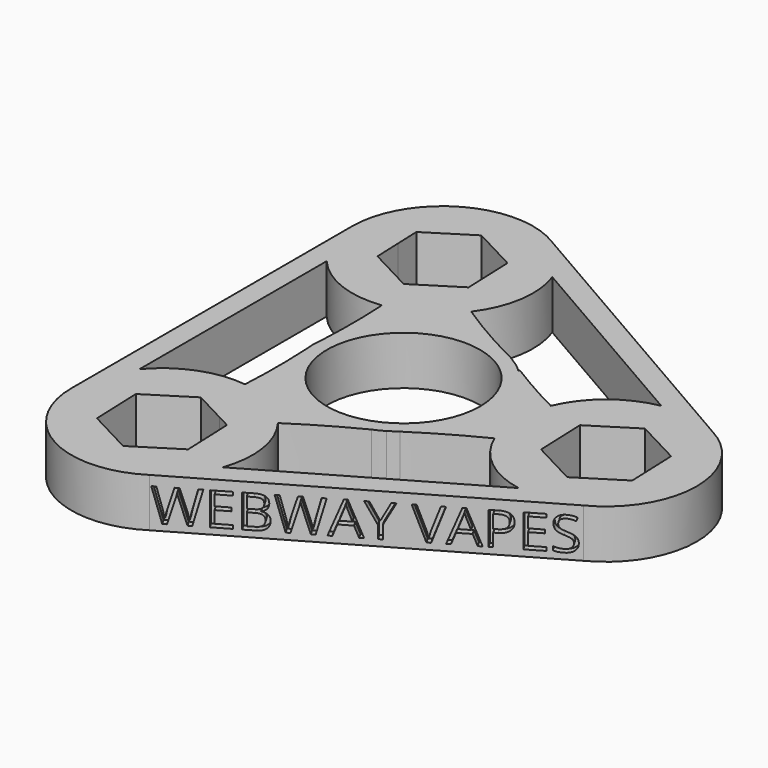
from build123d import *

# Parameters (mm, degrees)
F0_R         = 11
F1_DEPTH     = 7
F2_TEXT_SIZE = 6.7022724893
F3_DEPTH     = 1
F4_TEXT_SIZE = 6.5682270395
F5_DEPTH     = 1
F6_TEXT_SIZE = 6.5682270395
F7_DEPTH     = 1


# Not quite as in the source:
# - Text() gives the source's letters only with a copy of the font that has no kerning and outlines rounded to 1/6400 em; it was checked with that copy


with BuildPart() as f1:
    # F0 (on Top) → F1 (new body)
    with BuildSketch(Plane.XY):
        with BuildLine():
            ThreePointArc((-7.6287234995, 36.1940918561), (-20.8266237724, 36.5516209861), (-27.530946799, 25.1777715301))
            Line((-27.530946799, 25.1777715301), (-27.530946799, -25.1833324685))
            ThreePointArc((-27.530946799, -25.1833324685), (-20.7784207232, -36.5837302495), (-7.5357053272, -36.1408229088))
            Line((-7.5357053272, -36.1408229088), (35.0748929735, -11.5395825096))
            ThreePointArc((35.0748929735, -11.5395825096), (42.0829321515, -0.0578107695), (35.1723502351, 11.4828804138))
            Line((35.1723502351, 11.4828804138), (-7.6287234995, 36.1940918561))
        make_face()
        with Locations((-14.530946799, -25.1833324685)):
            Circle(F0_R, mode=Mode.SUBTRACT)
        with BuildLine():
            ThreePointArc((-12.9255685554, 12.277276939), (-12.7675398796, 6.9299853313), (-12.9033720663, 1.5820838534))
            ThreePointArc((-12.9033720663, 1.5820838534), (-6.4302872117, 11.2982921884), (5.2290918379, 11.9019577613))
            ThreePointArc((5.2290918379, 11.9019577613), (0.4581302885, 14.4888211029), (-4.1613203284, 17.3374369162))
            ThreePointArc((-4.1613203284, 17.3374369162), (-1.6796615961, 23.2170398726), (-2.2951140053, 29.5691717447))
            Line((-2.2951140053, 29.5691717447), (26.7681963735, 12.7894616739))
            ThreePointArc((26.7681963735, 12.7894616739), (20.9564789287, 10.144084315), (17.1054325569, 5.0506058502))
            ThreePointArc((17.1054325569, 5.0506058502), (13.0262022486, 7.2270838071), (9.054869709, 9.5947185056))
            Line((9.054869709, 9.5947185056), (8.948459988, 9.4300086873))
            ThreePointArc((8.948459988, 9.4300086873), (11.9442450545, 5.1317648113), (13, 0))
            ThreePointArc((13, 0), (11.62464331, -5.8195934493), (7.7895895515, -10.4077997011))
            ThreePointArc((7.7895895515, -10.4077997011), (12.3729190289, -7.6017999865), (17.104052334, -5.0528941141))
            ThreePointArc((17.104052334, -5.0528941141), (20.9524134175, -10.1463878699), (26.761439255, -12.7937980177))
            Line((26.761439255, -12.7937980177), (-2.2927959761, -29.5682685494))
            ThreePointArc((-2.2927959761, -29.5682685494), (-1.6817089539, -23.2092284187), (-4.173509012, -17.3269030958))
            ThreePointArc((-4.173509012, -17.3269030958), (0.3360289764, -14.5406855904), (4.9904853555, -12.0039600098))
            ThreePointArc((4.9904853555, -12.0039600098), (-6.6086120064, -11.1949206049), (-12.9210698593, -1.4303683763))
            ThreePointArc((-12.9210698593, -1.4303683763), (-12.7767748148, -6.8562127832), (-12.9349879797, -12.2816691863))
            ThreePointArc((-12.9349879797, -12.2816691863), (-19.2689540032, -13.0774955402), (-24.4604024316, -16.7925094551))
            Line((-24.4604024316, -16.7925094551), (-24.4604024316, 16.7869485168))
            ThreePointArc((-24.4604024316, 16.7869485168), (-19.2645342894, 13.0702057355), (-12.9255685554, 12.277276939))
        make_face(mode=Mode.SUBTRACT)
        with BuildLine():
            ThreePointArc((-25.530946799, 25.1777715301), (-14.530946799, 36.1777715301), (-3.530946799, 25.1777715301))
            ThreePointArc((-3.530946799, 25.1777715301), (-14.530946799, 14.1777715301), (-25.530946799, 25.1777715301))
        make_face(mode=Mode.SUBTRACT)
        with Locations((29.0830486264, -0.0027804692)):
            Circle(F0_R, mode=Mode.SUBTRACT)
        with BuildLine():
            ThreePointArc((-12.9033720663, 1.5820838534), (-12.9484673329, 0.7908453402), (-13, 0))
            ThreePointArc((-13, 0), (-12.9997736844, -0.0767082424), (-12.9990947455, -0.153413814))
            ThreePointArc((-12.9990947455, -0.153413814), (-12.9579854367, -0.7917629718), (-12.9210698593, -1.4303683763))
            ThreePointArc((-12.9210698593, -1.4303683763), (-6.6086120064, -11.1949206049), (4.9904853555, -12.0039600098))
            ThreePointArc((4.9904853555, -12.0039600098), (5.7761571729, -11.6462873189), (6.5363588729, -11.2372600168))
            ThreePointArc((6.5363588729, -11.2372600168), (7.1613741873, -10.8201123831), (7.7895895515, -10.4077997011))
            ThreePointArc((7.7895895515, -10.4077997011), (11.62464331, -5.8195934493), (13, 0))
            ThreePointArc((13, 0), (11.9442450545, 5.1317648113), (8.948459988, 9.4300086873))
            ThreePointArc((8.948459988, 9.4300086873), (8.4010552812, 9.9207998751), (7.8267807235, 10.3798604762))
            ThreePointArc((7.8267807235, 10.3798604762), (7.1580547417, 10.8183902406), (6.4929522165, 11.2623963486))
            ThreePointArc((6.4929522165, 11.2623963486), (6.4256273814, 11.3009430029), (6.3580737149, 11.3390872047))
            ThreePointArc((6.3580737149, 11.3390872047), (5.7926713707, 11.618694424), (5.2290918379, 11.9019577613))
            ThreePointArc((5.2290918379, 11.9019577613), (-6.4302872117, 11.2982921884), (-12.9033720663, 1.5820838534))
        make_face()
        with BuildLine():
            ThreePointArc((-11, 0), (0, 11), (11, 0))
            ThreePointArc((11, 0), (0, -11), (-11, 0))
        make_face(mode=Mode.SUBTRACT)
        with Locations((-14.530946799, -25.1833324685)):
            Circle(F0_R)
        Polygon((-21.0194197971, -21.7682114622), (-14.8176017496, -17.8565895173), (-10.2373305753, -20.2673540079), (-8.3291287516, -21.2717105235), (-8.042473801, -28.5984534747), (-14.2442918485, -32.5100754196), (-17.1564293953, -30.9773107596), (-20.7327648465, -29.0949544134), align=None, mode=Mode.SUBTRACT)
        with BuildLine():
            ThreePointArc((-25.530946799, 25.1777715301), (-14.530946799, 14.1777715301), (-3.530946799, 25.1777715301))
            ThreePointArc((-3.530946799, 25.1777715301), (-14.530946799, 36.1777715301), (-25.530946799, 25.1777715301))
        make_face()
        Polygon((-20.7457503175, 21.2642133583), (-20.8988662153, 25.1777715301), (-21.0324052681, 28.5909563095), (-14.8305872207, 32.5025782544), (-8.3421142227, 29.0874572482), (-8.0554592721, 21.760714297), (-14.2572773195, 17.8490923521), align=None, mode=Mode.SUBTRACT)
        with Locations((29.0830486264, -0.0027804692)):
            Circle(F0_R)
        Polygon((22.5864060711, 3.4226181715), (28.7882241186, 7.3342401164), (35.2766971166, 3.9191191101), (35.5633520672, -3.407623841), (29.3615340197, -7.319245786), (22.8730610217, -3.9041247797), align=None, mode=Mode.SUBTRACT)
    extrude(amount=F1_DEPTH)

    # F2 (on face) → F3 (cut)
    with BuildSketch(Plane(origin=(-27.530946799, 0, 0), x_dir=(0, -1, 0), z_dir=(-1, 0, 0))):
        with Locations((-24.9972394676, 0.9645518624)):
            Text('WEBWAY VAPES', F2_TEXT_SIZE, font='Open Sans', text_align=(TextAlign.LEFT, TextAlign.BOTTOM))
    extrude(amount=-F3_DEPTH, mode=Mode.SUBTRACT)

    # F4 (on face) → F5 (cut)
    with BuildSketch(Plane(origin=(13.7653206322, 23.8422347175, 0), x_dir=(-0.8660254038, 0.5, 0), z_dir=(0.5, 0.8660254038, 0))):
        with Locations((-24.7317176707, 0.8756756498)):
            Text('WEBWAY VAPES', F4_TEXT_SIZE, font='Open Sans', text_align=(TextAlign.LEFT, TextAlign.BOTTOM))
    extrude(amount=-F5_DEPTH, mode=Mode.SUBTRACT)

    # F6 (on face) → F7 (cut)
    with BuildSketch(Plane(origin=(13.7655090446, -23.8425610572, 0), x_dir=(0.8660254038, 0.5, 0), z_dir=(0.5, -0.8660254038, 0))):
        with Locations((-24.5, 0.9152976125)):
            Text('WEBWAY VAPES', F6_TEXT_SIZE, font='Open Sans', text_align=(TextAlign.LEFT, TextAlign.BOTTOM))
    extrude(amount=-F7_DEPTH, mode=Mode.SUBTRACT)


solid = f1.part
